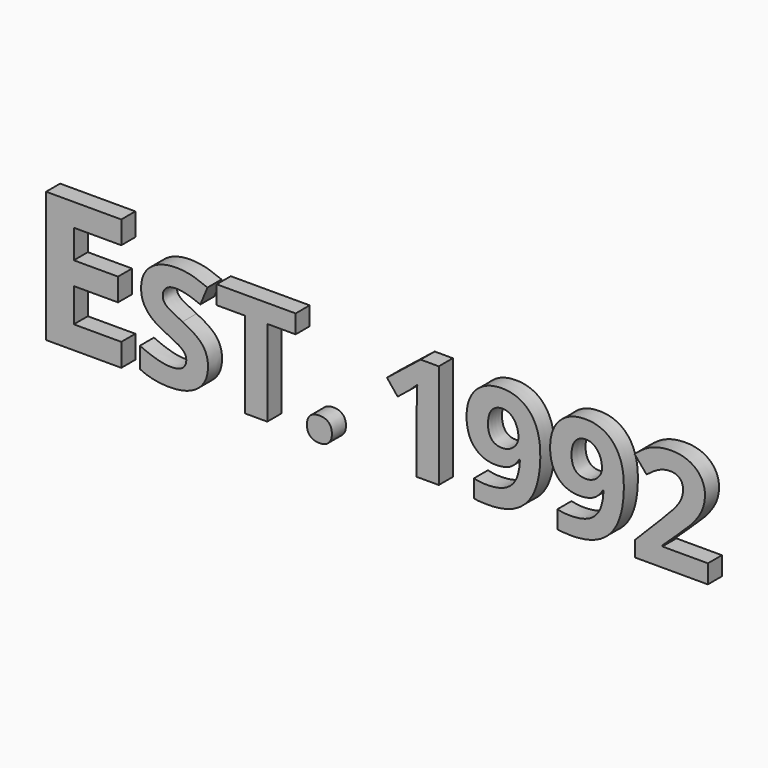
from build123d import *

# Parameters (mm, degrees)
F0_TEXT_SIZE   = 208.3333333333
F0_TEXT_SIZE_2 = 166.6666666667
F1_DEPTH       = 20


# Not quite as in the source:
# - Text() gives the source's letters only with a copy of the font that has no kerning and outlines rounded to 1/6400 em; it was checked with that copy


with BuildPart() as f1:
    # F0 (on Front) → F1 (new body)
    with BuildSketch(Plane.XZ):
        with Locations((-504.6014469057, -75.0842376246)):
            Text('E', F0_TEXT_SIZE, font='Open Sans', font_style=FontStyle.BOLD, text_align=(TextAlign.LEFT, TextAlign.BOTTOM))
        with Locations((-386.7303531557, -74.9765003473)):
            Text('ST. 1992', F0_TEXT_SIZE_2, font='Open Sans', font_style=FontStyle.BOLD, text_align=(TextAlign.LEFT, TextAlign.BOTTOM))
    extrude(amount=F1_DEPTH)


solid = f1.part
